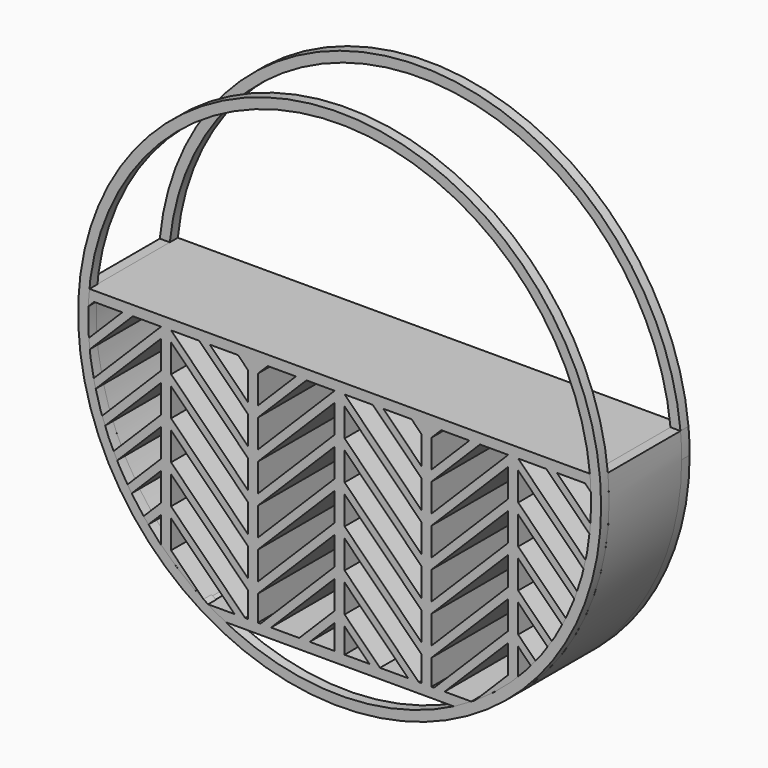
from build123d import *
from build123d import SkipClean  # not in build123d's __all__

# Parameters (mm, degrees)
F1_R     = 66.675
F1_R_2   = 64.135
F2_DEPTH = 2.54
F0_W     = 1.27
F0_H     = 2.54
F0_W_2   = 2.54
F3_DEPTH = 28.2045833333
F4_DEPTH = 25.6645833333
F5_START = 25.6645833333
F5_DEPTH = 2.54


with BuildPart() as f2:
    # F1 (on Front) → F2 (new body)
    with BuildSketch(Plane.XZ):
        Circle(F1_R)
        Circle(F1_R_2, mode=Mode.SUBTRACT)
    extrude(amount=F2_DEPTH)

    # F0 (on Front) → F3 (join)
    with BuildSketch(Plane.XZ):
        Polygon((42.9779534994, 6.35), (23.3939767497, 6.35), (23.3939767497, 3.81), (25.9154668694, 3.81), (33.0996717663, 3.81), (35.7937486026, 3.81), (42.9779534994, 3.81), align=None)
        with BuildLine():
            ThreePointArc((64.021731662, 3.81), (63.9334156596, 5.0810025681), (63.819869359, 6.35))
            Line((63.819869359, 6.35), (45.5179534994, 6.35))
            Line((45.5179534994, 6.35), (45.5179534994, 3.81))
            Line((45.5179534994, 3.81), (52.7021583963, 3.81))
            Line((52.7021583963, 3.81), (55.3962352326, 3.81))
            Line((55.3962352326, 3.81), (62.5804401295, 3.81))
            Line((62.5804401295, 3.81), (64.021731662, 3.81))
        make_face()
        Polygon((20.8539767497, 6.35), (1.27, 6.35), (1.27, 3.81), (8.4542048969, 3.81), (11.1482817332, 3.81), (18.33248663, 3.81), (20.8539767497, 3.81), align=None)
        Polygon((-1.27, 6.35), (-20.8539767497, 6.35), (-20.8539767497, 3.81), (-18.33248663, 3.81), (-11.1482817332, 3.81), (-8.4542048969, 3.81), (-1.27, 3.81), align=None)
        Polygon((-23.3939767497, 6.35), (-42.9779534994, 6.35), (-42.9779534994, 3.81), (-35.7937486026, 3.81), (-33.0996717663, 3.81), (-25.9154668694, 3.81), (-23.3939767497, 3.81), align=None)
        with BuildLine():
            Line((-45.5179534994, 6.35), (-63.819869359, 6.35))
            ThreePointArc((-63.819869359, 6.35), (-63.9334156596, 5.0810025681), (-64.021731662, 3.81))
            Line((-64.021731662, 3.81), (-62.5804401295, 3.81))
            Line((-62.5804401295, 3.81), (-55.3962352326, 3.81))
            Line((-55.3962352326, 3.81), (-52.7021583963, 3.81))
            Line((-52.7021583963, 3.81), (-45.5179534994, 3.81))
            Line((-45.5179534994, 3.81), (-45.5179534994, 6.35))
        make_face()
        Polygon((-44.2479534994, 6.35), (-45.5179534994, 6.35), (-45.5179534994, 3.81), (-42.9779534994, 3.81), (-42.9779534994, 6.35), align=None)
        with BuildLine():
            Line((-42.9779534994, 3.81), (-45.5179534994, 3.81))
            Line((-45.5179534994, 3.81), (-45.5179534994, 1.1159231637))
            Line((-45.5179534994, 1.1159231637), (-45.5179534994, -6.0682817332))
            Line((-45.5179534994, -6.0682817332), (-45.5179534994, -8.7910953891))
            Line((-45.5179534994, -8.7910953891), (-45.5179534994, -15.9753002859))
            Line((-45.5179534994, -15.9753002859), (-45.5179534994, -18.6693771223))
            Line((-45.5179534994, -18.6693771223), (-45.5179534994, -25.8535820191))
            Line((-45.5179534994, -25.8535820191), (-45.5179534994, -28.5476588554))
            Line((-45.5179534994, -28.5476588554), (-45.5179534994, -35.7318637523))
            Line((-45.5179534994, -35.7318637523), (-45.5179534994, -38.4259405886))
            Line((-45.5179534994, -38.4259405886), (-45.5179534994, -45.1820111795))
            ThreePointArc((-45.5179534994, -45.1820111795), (-44.2645294741, -46.4106631652), (-42.9779534994, -47.6045558534))
            Line((-42.9779534994, -47.6045558534), (-42.9779534994, -45.5814086659))
            Line((-42.9779534994, -45.5814086659), (-42.9779534994, -38.397203769))
            Line((-42.9779534994, -38.397203769), (-42.9779534994, -35.7031269327))
            Line((-42.9779534994, -35.7031269327), (-42.9779534994, -28.5189220358))
            Line((-42.9779534994, -28.5189220358), (-42.9779534994, -25.8248451995))
            Line((-42.9779534994, -25.8248451995), (-42.9779534994, -18.6406403027))
            Line((-42.9779534994, -18.6406403027), (-42.9779534994, -15.9465634664))
            Line((-42.9779534994, -15.9465634664), (-42.9779534994, -8.7623585695))
            Line((-42.9779534994, -8.7623585695), (-42.9779534994, -6.0682817332))
            Line((-42.9779534994, -6.0682817332), (-42.9779534994, 1.1159231637))
            Line((-42.9779534994, 1.1159231637), (-42.9779534994, 3.81))
        make_face()
        Polygon((-22.1239767497, 6.35), (-23.3939767497, 6.35), (-23.3939767497, 3.81), (-20.8539767497, 3.81), (-20.8539767497, 6.35), align=None)
        Polygon((-23.3939767497, -8.5897718529), (-23.3939767497, -15.7739767497), (-23.3939767497, -18.468053586), (-23.3939767497, -25.6522584829), (-23.3939767497, -28.3463353192), (-23.3939767497, -35.5305402161), (-23.3939767497, -38.2246170524), (-23.3939767497, -45.4088219492), (-23.3939767497, -48.1028987856), (-23.3939767497, -54.61), (-20.8539767497, -54.61), (-20.8539767497, -48.1028987856), (-20.8539767497, -45.4088219492), (-20.8539767497, -38.2246170524), (-20.8539767497, -35.5305402161), (-20.8539767497, -28.3463353192), (-20.8539767497, -25.6522584829), (-20.8539767497, -18.468053586), (-20.8539767497, -15.7739767497), (-20.8539767497, -8.5897718529), (-20.8539767497, -5.8956950165), (-20.8539767497, 1.2885098803), (-20.8539767497, 3.81), (-23.3939767497, 3.81), (-23.3939767497, 1.2885098803), (-23.3939767497, -5.8956950165), align=None)
        with Locations((-0.635, 5.08)):
            Rectangle(F0_W, F0_H)
        Polygon((-1.27, -48.2754855022), (-1.27, -54.61), (0, -54.61), (0, 3.81), (-1.27, 3.81), (-1.27, 1.1159231637), (-1.27, -6.0682817332), (-1.27, -8.7623585695), (-1.27, -15.9465634664), (-1.27, -18.6406403027), (-1.27, -25.8248451995), (-1.27, -28.5189220358), (-1.27, -35.7031269327), (-1.27, -38.397203769), (-1.27, -45.5814086659), align=None)
        with Locations((0.635, 5.08)):
            Rectangle(F0_W, F0_H)
        Polygon((0, 3.81), (0, -54.61), (1.27, -54.61), (1.27, -48.2754855022), (1.27, -45.5814086659), (1.27, -38.397203769), (1.27, -35.7031269327), (1.27, -28.5189220358), (1.27, -25.8248451995), (1.27, -18.6406403027), (1.27, -15.9465634664), (1.27, -8.7623585695), (1.27, -6.0682817332), (1.27, 1.1159231637), (1.27, 3.81), align=None)
        Polygon((22.1239767497, 6.35), (20.8539767497, 6.35), (20.8539767497, 3.81), (23.3939767497, 3.81), (23.3939767497, 6.35), align=None)
        Polygon((20.8539767497, -48.1028987856), (20.8539767497, -54.61), (23.3939767497, -54.61), (23.3939767497, -48.1028987856), (23.3939767497, -45.4088219492), (23.3939767497, -38.2246170524), (23.3939767497, -35.5305402161), (23.3939767497, -28.3463353192), (23.3939767497, -25.6522584829), (23.3939767497, -18.468053586), (23.3939767497, -15.7739767497), (23.3939767497, -8.5897718529), (23.3939767497, -5.8956950165), (23.3939767497, 1.2885098803), (23.3939767497, 3.81), (20.8539767497, 3.81), (20.8539767497, 1.2885098803), (20.8539767497, -5.8956950165), (20.8539767497, -8.5897718529), (20.8539767497, -15.7739767497), (20.8539767497, -18.468053586), (20.8539767497, -25.6522584829), (20.8539767497, -28.3463353192), (20.8539767497, -35.5305402161), (20.8539767497, -38.2246170524), (20.8539767497, -45.4088219492), align=None)
        Polygon((44.2479534994, 6.35), (42.9779534994, 6.35), (42.9779534994, 3.81), (45.5179534994, 3.81), (45.5179534994, 6.35), align=None)
        with BuildLine():
            Line((42.9779534994, -25.8248451995), (42.9779534994, -28.5189220358))
            Line((42.9779534994, -28.5189220358), (42.9779534994, -35.7031269327))
            Line((42.9779534994, -35.7031269327), (42.9779534994, -38.397203769))
            Line((42.9779534994, -38.397203769), (42.9779534994, -45.5814086659))
            Line((42.9779534994, -45.5814086659), (42.9779534994, -47.6045558534))
            ThreePointArc((42.9779534994, -47.6045558534), (44.2645294741, -46.4106631652), (45.5179534994, -45.1820111795))
            Line((45.5179534994, -45.1820111795), (45.5179534994, -38.397203769))
            Line((45.5179534994, -38.397203769), (45.5179534994, -35.7031269327))
            Line((45.5179534994, -35.7031269327), (45.5179534994, -28.5189220358))
            Line((45.5179534994, -28.5189220358), (45.5179534994, -25.8248451995))
            Line((45.5179534994, -25.8248451995), (45.5179534994, -18.6406403027))
            Line((45.5179534994, -18.6406403027), (45.5179534994, -15.9465634664))
            Line((45.5179534994, -15.9465634664), (45.5179534994, -8.7623585695))
            Line((45.5179534994, -8.7623585695), (45.5179534994, -6.0682817332))
            Line((45.5179534994, -6.0682817332), (45.5179534994, 1.1159231637))
            Line((45.5179534994, 1.1159231637), (45.5179534994, 3.81))
            Line((45.5179534994, 3.81), (42.9779534994, 3.81))
            Line((42.9779534994, 3.81), (42.9779534994, 1.1159231637))
            Line((42.9779534994, 1.1159231637), (42.9779534994, -6.0682817332))
            Line((42.9779534994, -6.0682817332), (42.9779534994, -8.7623585695))
            Line((42.9779534994, -8.7623585695), (42.9779534994, -15.9465634664))
            Line((42.9779534994, -15.9465634664), (42.9779534994, -18.6406403027))
            Line((42.9779534994, -18.6406403027), (42.9779534994, -25.8248451995))
        make_face()
        with BuildLine():
            ThreePointArc((64.093868536, 2.2965715934), (64.0622694721, 3.0534988273), (64.021731662, 3.81))
            Line((64.021731662, 3.81), (62.5804401295, 3.81))
            Line((62.5804401295, 3.81), (64.093868536, 2.2965715934))
        make_face()
        with BuildLine():
            Line((55.3962352326, 3.81), (52.7021583963, 3.81))
            Line((52.7021583963, 3.81), (63.7278017507, -7.2156433544))
            ThreePointArc((63.7278017507, -7.2156433544), (63.8551182502, -5.985156494), (63.9586781545, -4.7524429219))
            Line((63.9586781545, -4.7524429219), (55.3962352326, 3.81))
        make_face()
        with BuildLine():
            Line((62.721004529, -13.3930510295), (45.5179534994, 3.81))
            Line((45.5179534994, 3.81), (45.5179534994, 1.1159231637))
            Line((45.5179534994, 1.1159231637), (62.2138469406, -15.5799702775))
            ThreePointArc((62.2138469406, -15.5799702775), (62.4769952213, -14.4887298656), (62.721004529, -13.3930510295))
        make_face()
        with BuildLine():
            Line((60.5608489339, -21.1111771676), (45.5179534994, -6.0682817332))
            Line((45.5179534994, -6.0682817332), (45.5179534994, -8.7623585695))
            Line((45.5179534994, -8.7623585695), (59.837484787, -23.081889857))
            ThreePointArc((59.837484787, -23.081889857), (60.2072306108, -22.0994933694), (60.5608489339, -21.1111771676))
        make_face()
        with BuildLine():
            Line((57.6579743515, -28.0865843184), (45.5179534994, -15.9465634664))
            Line((45.5179534994, -15.9465634664), (45.5179534994, -18.6406403027))
            Line((45.5179534994, -18.6406403027), (56.7520681626, -29.8747549658))
            ThreePointArc((56.7520681626, -29.8747549658), (57.2120078794, -28.984209139), (57.6579743515, -28.0865843184))
        make_face()
        with BuildLine():
            Line((45.5179534994, -28.5189220358), (53.0462029804, -36.0471715168))
            ThreePointArc((53.0462029804, -36.0471715168), (53.5867591338, -35.2385792922), (54.1149908049, -34.421882505))
            Line((54.1149908049, -34.421882505), (45.5179534994, -25.8248451995))
            Line((45.5179534994, -25.8248451995), (45.5179534994, -28.5189220358))
        make_face()
        with BuildLine():
            Line((45.5179534994, -38.397203769), (48.7706927508, -41.6499430204))
            ThreePointArc((48.7706927508, -41.6499430204), (49.3865441375, -40.9178137631), (49.9914060898, -40.176579523))
            Line((49.9914060898, -40.176579523), (45.5179534994, -35.7031269327))
            Line((45.5179534994, -35.7031269327), (45.5179534994, -38.397203769))
        make_face()
        with BuildLine():
            Line((42.9779534994, -45.5814086659), (34.4838168677, -54.0755452976))
            ThreePointArc((34.4838168677, -54.0755452976), (38.8657933561, -51.0171376284), (42.9779534994, -47.6045558534))
            Line((42.9779534994, -47.6045558534), (42.9779534994, -45.5814086659))
        make_face()
        Polygon((42.9779534994, -35.7031269327), (24.0710804321, -54.61), (26.7651572685, -54.61), (42.9779534994, -38.397203769), align=None)
        Polygon((23.3939767497, -45.4088219492), (23.3939767497, -48.1028987856), (42.9779534994, -28.5189220358), (42.9779534994, -25.8248451995), align=None)
        Polygon((23.3939767497, -35.5305402161), (23.3939767497, -38.2246170524), (42.9779534994, -18.6406403027), (42.9779534994, -15.9465634664), align=None)
        Polygon((23.3939767497, -25.6522584829), (23.3939767497, -28.3463353192), (42.9779534994, -8.7623585695), (42.9779534994, -6.0682817332), align=None)
        Polygon((42.9779534994, 1.1159231637), (42.9779534994, 3.81), (23.3939767497, -15.7739767497), (23.3939767497, -18.468053586), align=None)
        Polygon((33.0996717663, 3.81), (23.3939767497, -5.8956950165), (23.3939767497, -8.5897718529), (35.7937486026, 3.81), align=None)
        Polygon((25.9154668694, 3.81), (23.3939767497, 3.81), (23.3939767497, 1.2885098803), align=None)
        Polygon((20.8539767497, 1.2885098803), (20.8539767497, 3.81), (18.33248663, 3.81), align=None)
        Polygon((11.1482817332, 3.81), (8.4542048969, 3.81), (20.8539767497, -8.5897718529), (20.8539767497, -5.8956950165), align=None)
        Polygon((20.8539767497, -15.7739767497), (1.27, 3.81), (1.27, 1.1159231637), (20.8539767497, -18.468053586), align=None)
        Polygon((20.8539767497, -25.6522584829), (1.27, -6.0682817332), (1.27, -8.7623585695), (20.8539767497, -28.3463353192), align=None)
        Polygon((1.27, -18.6406403027), (20.8539767497, -38.2246170524), (20.8539767497, -35.5305402161), (1.27, -15.9465634664), align=None)
        Polygon((1.27, -28.5189220358), (20.8539767497, -48.1028987856), (20.8539767497, -45.4088219492), (1.27, -25.8248451995), align=None)
        Polygon((17.482796231, -54.61), (20.1768730673, -54.61), (1.27, -35.7031269327), (1.27, -38.397203769), align=None)
        Polygon((1.27, -45.5814086659), (1.27, -48.2754855022), (7.6045144978, -54.61), (10.2985913341, -54.61), align=None)
        Polygon((-7.6045144978, -54.61), (-1.27, -48.2754855022), (-1.27, -45.5814086659), (-10.2985913341, -54.61), align=None)
        Polygon((-1.27, -35.7031269327), (-20.1768730673, -54.61), (-17.482796231, -54.61), (-1.27, -38.397203769), align=None)
        Polygon((-20.8539767497, -45.4088219492), (-20.8539767497, -48.1028987856), (-1.27, -28.5189220358), (-1.27, -25.8248451995), align=None)
        Polygon((-20.8539767497, -35.5305402161), (-20.8539767497, -38.2246170524), (-1.27, -18.6406403027), (-1.27, -15.9465634664), align=None)
        Polygon((-1.27, -8.7623585695), (-1.27, -6.0682817332), (-20.8539767497, -25.6522584829), (-20.8539767497, -28.3463353192), align=None)
        Polygon((-1.27, 1.1159231637), (-1.27, 3.81), (-20.8539767497, -15.7739767497), (-20.8539767497, -18.468053586), align=None)
        Polygon((-11.1482817332, 3.81), (-20.8539767497, -5.8956950165), (-20.8539767497, -8.5897718529), (-8.4542048969, 3.81), align=None)
        Polygon((-18.33248663, 3.81), (-20.8539767497, 3.81), (-20.8539767497, 1.2885098803), align=None)
        Polygon((-23.3939767497, 1.2885098803), (-23.3939767497, 3.81), (-25.9154668694, 3.81), align=None)
        Polygon((-33.0996717663, 3.81), (-35.7937486026, 3.81), (-23.3939767497, -8.5897718529), (-23.3939767497, -5.8956950165), align=None)
        Polygon((-23.3939767497, -15.7739767497), (-42.9779534994, 3.81), (-42.9779534994, 1.1159231637), (-23.3939767497, -18.468053586), align=None)
        Polygon((-23.3939767497, -25.6522584829), (-42.9779534994, -6.0682817332), (-42.9779534994, -8.7623585695), (-23.3939767497, -28.3463353192), align=None)
        Polygon((-23.3939767497, -35.5305402161), (-42.9779534994, -15.9465634664), (-42.9779534994, -18.6406403027), (-23.3939767497, -38.2246170524), align=None)
        Polygon((-42.9779534994, -28.5189220358), (-23.3939767497, -48.1028987856), (-23.3939767497, -45.4088219492), (-42.9779534994, -25.8248451995), align=None)
        Polygon((-42.9779534994, -38.397203769), (-26.7651572685, -54.61), (-24.0710804321, -54.61), (-42.9779534994, -35.7031269327), align=None)
        with BuildLine():
            ThreePointArc((-42.9779534994, -47.6045558534), (-38.8657933561, -51.0171376284), (-34.4838168677, -54.0755452976))
            Line((-34.4838168677, -54.0755452976), (-42.9779534994, -45.5814086659))
            Line((-42.9779534994, -45.5814086659), (-42.9779534994, -47.6045558534))
        make_face()
        with BuildLine():
            ThreePointArc((-49.9785993713, -40.1925096241), (-49.3735194143, -40.933529113), (-48.7574535758, -41.665440665))
            Line((-48.7574535758, -41.665440665), (-45.5179534994, -38.4259405886))
            Line((-45.5179534994, -38.4259405886), (-45.5179534994, -35.7318637523))
            Line((-45.5179534994, -35.7318637523), (-49.9785993713, -40.1925096241))
        make_face()
        with BuildLine():
            Line((-45.5179534994, -28.5476588554), (-45.5179534994, -25.8535820191))
            Line((-45.5179534994, -25.8535820191), (-54.1038158894, -34.4394444091))
            ThreePointArc((-54.1038158894, -34.4394444091), (-53.5753548837, -35.2559154481), (-53.0345736643, -36.0642790203))
            Line((-53.0345736643, -36.0642790203), (-45.5179534994, -28.5476588554))
        make_face()
        with BuildLine():
            Line((-45.5179534994, -18.6693771223), (-45.5179534994, -15.9753002859))
            Line((-45.5179534994, -15.9753002859), (-57.6485585927, -28.1059053792))
            ThreePointArc((-57.6485585927, -28.1059053792), (-57.2023407946, -29.0032831352), (-56.742155162, -29.8935787849))
            Line((-56.742155162, -29.8935787849), (-45.5179534994, -18.6693771223))
        make_face()
        with BuildLine():
            Line((-45.5179534994, -8.7910953891), (-45.5179534994, -6.0682817332))
            Line((-45.5179534994, -6.0682817332), (-60.5608489339, -21.1111771676))
            ThreePointArc((-60.5608489339, -21.1111771676), (-60.2034005634, -22.1099250476), (-59.8294824704, -23.1026243601))
            Line((-59.8294824704, -23.1026243601), (-45.5179534994, -8.7910953891))
        make_face()
        with BuildLine():
            Line((-45.5179534994, 1.1159231637), (-45.5179534994, 3.81))
            Line((-45.5179534994, 3.81), (-62.721004529, -13.3930510295))
            ThreePointArc((-62.721004529, -13.3930510295), (-62.4769952213, -14.4887298656), (-62.2138469406, -15.5799702775))
            Line((-62.2138469406, -15.5799702775), (-45.5179534994, 1.1159231637))
        make_face()
        with BuildLine():
            Line((-63.7278017507, -7.2156433544), (-52.7021583963, 3.81))
            Line((-52.7021583963, 3.81), (-55.3962352326, 3.81))
            Line((-55.3962352326, 3.81), (-63.9586781545, -4.7524429219))
            ThreePointArc((-63.9586781545, -4.7524429219), (-63.8551182502, -5.985156494), (-63.7278017507, -7.2156433544))
        make_face()
        with BuildLine():
            Line((-62.5804401295, 3.81), (-64.021731662, 3.81))
            ThreePointArc((-64.021731662, 3.81), (-64.0622694721, 3.0534988273), (-64.093868536, 2.2965715934))
            Line((-64.093868536, 2.2965715934), (-62.5804401295, 3.81))
        make_face()
        with BuildLine():
            ThreePointArc((-33.6310291992, -54.61), (-31.3943544851, -55.9257787739), (-29.1062832564, -57.15))
            Line((-29.1062832564, -57.15), (-23.3939767497, -57.15))
            Line((-23.3939767497, -57.15), (-23.3939767497, -54.61))
            Line((-23.3939767497, -54.61), (-24.0710804321, -54.61))
            Line((-24.0710804321, -54.61), (-26.7651572685, -54.61))
            Line((-26.7651572685, -54.61), (-33.6310291992, -54.61))
        make_face()
        with Locations((-22.1239767497, -55.88)):
            Rectangle(F0_W_2, F0_H)
        Polygon((-20.8539767497, -54.61), (-20.8539767497, -57.15), (-1.27, -57.15), (-1.27, -54.61), (-7.6045144978, -54.61), (-10.2985913341, -54.61), (-17.482796231, -54.61), (-20.1768730673, -54.61), align=None)
        with Locations((-0.635, -55.88)):
            Rectangle(F0_W, F0_H)
        with Locations((0.635, -55.88)):
            Rectangle(F0_W, F0_H)
        Polygon((1.27, -54.61), (1.27, -57.15), (20.8539767497, -57.15), (20.8539767497, -54.61), (20.1768730673, -54.61), (17.482796231, -54.61), (10.2985913341, -54.61), (7.6045144978, -54.61), align=None)
        with BuildLine():
            Line((23.3939767497, -54.61), (23.3939767497, -57.15))
            Line((23.3939767497, -57.15), (29.1062832564, -57.15))
            ThreePointArc((29.1062832564, -57.15), (31.3943544851, -55.9257787739), (33.6310291992, -54.61))
            Line((33.6310291992, -54.61), (26.7651572685, -54.61))
            Line((26.7651572685, -54.61), (24.0710804321, -54.61))
            Line((24.0710804321, -54.61), (23.3939767497, -54.61))
        make_face()
        with Locations((22.1239767497, -55.88)):
            Rectangle(F0_W_2, F0_H)
    extrude(amount=F3_DEPTH)

    # F0 (on Front) → F4 (join)
    with BuildSketch(Plane.XZ):
        with BuildLine():
            Line((-64.021731662, 3.81), (-66.5660538488, 3.81))
            ThreePointArc((-66.5660538488, 3.81), (-58.9464454034, -31.1588221745), (-34.3428758988, -57.15))
            Line((-34.3428758988, -57.15), (-29.1062832564, -57.15))
            ThreePointArc((-29.1062832564, -57.15), (-31.3943544851, -55.9257787739), (-33.6310291992, -54.61))
            ThreePointArc((-33.6310291992, -54.61), (-34.0584714005, -54.3444454463), (-34.4838168677, -54.0755452976))
            ThreePointArc((-34.4838168677, -54.0755452976), (-38.8657933561, -51.0171376284), (-42.9779534994, -47.6045558534))
            ThreePointArc((-42.9779534994, -47.6045558534), (-44.2645294741, -46.4106631652), (-45.5179534994, -45.1820111795))
            ThreePointArc((-45.5179534994, -45.1820111795), (-47.1704850711, -43.4539246001), (-48.7574535758, -41.665440665))
            ThreePointArc((-48.7574535758, -41.665440665), (-49.3735194143, -40.933529113), (-49.9785993713, -40.1925096241))
            ThreePointArc((-49.9785993713, -40.1925096241), (-51.5479294123, -38.1589989165), (-53.0345736643, -36.0642790203))
            ThreePointArc((-53.0345736643, -36.0642790203), (-53.5753548837, -35.2559154481), (-54.1038158894, -34.4394444091))
            ThreePointArc((-54.1038158894, -34.4394444091), (-55.4695731744, -32.1935502368), (-56.742155162, -29.8935787849))
            ThreePointArc((-56.742155162, -29.8935787849), (-57.2023407946, -29.0032831352), (-57.6485585927, -28.1059053792))
            ThreePointArc((-57.6485585927, -28.1059053792), (-58.792267674, -25.6274752318), (-59.8294824704, -23.1026243601))
            ThreePointArc((-59.8294824704, -23.1026243601), (-60.2034005634, -22.1099250476), (-60.5608489339, -21.1111771676))
            ThreePointArc((-60.5608489339, -21.1111771676), (-61.4496139059, -18.3641818716), (-62.2138469406, -15.5799702775))
            ThreePointArc((-62.2138469406, -15.5799702775), (-62.4769952213, -14.4887298656), (-62.721004529, -13.3930510295))
            ThreePointArc((-62.721004529, -13.3930510295), (-63.299804453, -10.3166361385), (-63.7278017507, -7.2156433544))
            ThreePointArc((-63.7278017507, -7.2156433544), (-63.8551182502, -5.985156494), (-63.9586781545, -4.7524429219))
            ThreePointArc((-63.9586781545, -4.7524429219), (-64.1232082003, -1.2297947411), (-64.093868536, 2.2965715934))
            ThreePointArc((-64.093868536, 2.2965715934), (-64.0622694721, 3.0534988273), (-64.021731662, 3.81))
        make_face()
        with BuildLine():
            Line((-63.819869359, 6.35), (-66.3719302492, 6.35))
            ThreePointArc((-66.3719302492, 6.35), (-66.4811236669, 5.0809271785), (-66.5660538488, 3.81))
            Line((-66.5660538488, 3.81), (-64.021731662, 3.81))
            ThreePointArc((-64.021731662, 3.81), (-63.9334156596, 5.0810025681), (-63.819869359, 6.35))
        make_face()
        with BuildLine():
            ThreePointArc((33.6310291992, -54.61), (31.3943544851, -55.9257787739), (29.1062832564, -57.15))
            Line((29.1062832564, -57.15), (34.3428758988, -57.15))
            ThreePointArc((34.3428758988, -57.15), (59.5309209097, -30.0270724621), (66.3719302492, 6.35))
            Line((66.3719302492, 6.35), (63.819869359, 6.35))
            ThreePointArc((63.819869359, 6.35), (63.9334156596, 5.0810025681), (64.021731662, 3.81))
            ThreePointArc((64.021731662, 3.81), (64.0622694721, 3.0534988273), (64.093868536, 2.2965715934))
            ThreePointArc((64.093868536, 2.2965715934), (64.1232082003, -1.2297947411), (63.9586781545, -4.7524429219))
            ThreePointArc((63.9586781545, -4.7524429219), (63.8551182502, -5.985156494), (63.7278017507, -7.2156433544))
            ThreePointArc((63.7278017507, -7.2156433544), (63.299804453, -10.3166361385), (62.721004529, -13.3930510295))
            ThreePointArc((62.721004529, -13.3930510295), (62.4769952213, -14.4887298656), (62.2138469406, -15.5799702775))
            ThreePointArc((62.2138469406, -15.5799702775), (61.4496139059, -18.3641818716), (60.5608489339, -21.1111771676))
            ThreePointArc((60.5608489339, -21.1111771676), (60.2072306108, -22.0994933694), (59.837484787, -23.081889857))
            ThreePointArc((59.837484787, -23.081889857), (58.8009988963, -25.6074355177), (57.6579743515, -28.0865843184))
            ThreePointArc((57.6579743515, -28.0865843184), (57.2120078794, -28.984209139), (56.7520681626, -29.8747549658))
            ThreePointArc((56.7520681626, -29.8747549658), (55.4801341314, -32.1753468009), (54.1149908049, -34.421882505))
            ThreePointArc((54.1149908049, -34.421882505), (53.5867591338, -35.2385792922), (53.0462029804, -36.0471715168))
            ThreePointArc((53.0462029804, -36.0471715168), (51.5601612036, -38.1424697897), (49.9914060898, -40.176579523))
            ThreePointArc((49.9914060898, -40.176579523), (49.3865441375, -40.9178137631), (48.7706927508, -41.6499430204))
            ThreePointArc((48.7706927508, -41.6499430204), (47.1773894922, -43.4464284574), (45.5179534994, -45.1820111795))
            ThreePointArc((45.5179534994, -45.1820111795), (44.2645294741, -46.4106631652), (42.9779534994, -47.6045558534))
            ThreePointArc((42.9779534994, -47.6045558534), (38.8657933561, -51.0171376284), (34.4838168677, -54.0755452976))
            ThreePointArc((34.4838168677, -54.0755452976), (34.0584714005, -54.3444454463), (33.6310291992, -54.61))
        make_face()
    with SkipClean():  # cleaning this boolean's faces spoils the solid; the shape is the same uncleaned
        extrude(amount=F4_DEPTH)


with BuildPart() as f5:
    # F1 (on Front) → F5 (new body)
    with BuildSketch(Plane.XZ.offset(F5_START)):
        Circle(F1_R)
        Circle(F1_R_2, mode=Mode.SUBTRACT)
    extrude(amount=F5_DEPTH)


solid = Compound([f2.part, f5.part])
